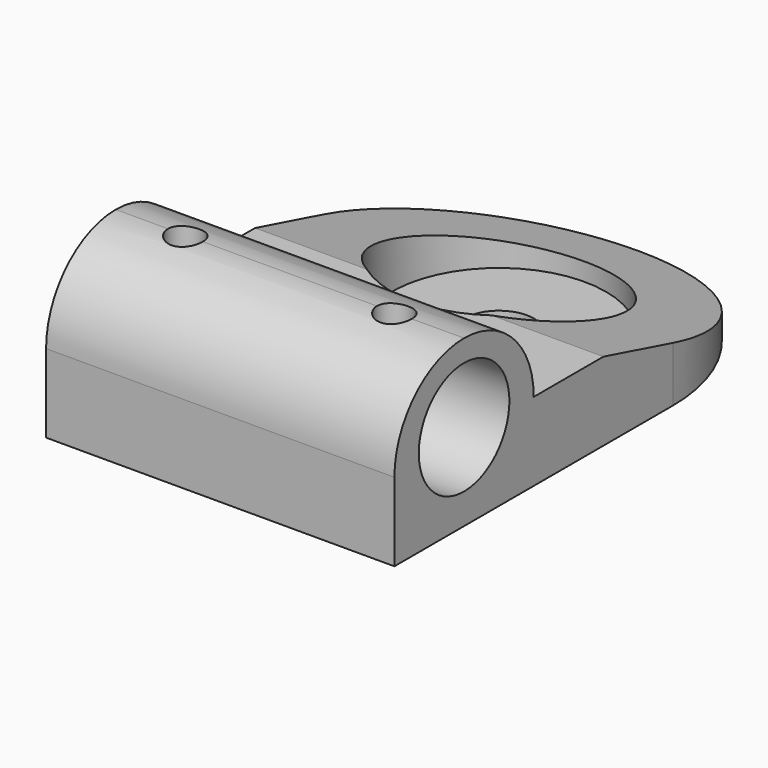
from build123d import *

# Parameters (mm, degrees)
F0_W         = 20
F0_H         = 30
F0_R         = 6.15
F1_DEPTH     = 4
F1_FACE_W    = 20
F1_FACE_H    = 30
F1_FACE_R    = 6.15
F0_R_2       = 2
F2_DEPTH     = 0.5
F3_W         = 20
F3_H         = 10
F4_DEPTH     = 5
F5_R         = 3.25
F6_DEPTH     = 25
F7_T1_DEPTH  = 97.9025398997
F8_R         = 9.99999
F9_R         = 1
F10_DEPTH    = 25
F11_T1_DEPTH = 45


# Not quite as in the source:
# - a fillet or chamfer that OpenCascade refuses, or shapes differently, is made with other operations: its cross-section is extruded or revolved along the edge and cut away or added
# - a fillet or chamfer is up to 0.001 mm smaller than in the source, because OpenCascade refuses the exact size
# - a feature names something its author has since deleted; it is built from what else it names


with BuildPart() as f1:
    # F0 (on Top) → F1 (new body)
    with BuildSketch(Plane.XY):
        with Locations((10, 15)):
            Rectangle(F0_W, F0_H)
        with Locations((10, 20)):
            Circle(F0_R, mode=Mode.SUBTRACT)
    extrude(amount=F1_DEPTH)

    # F1_face (on face) + F0 (on Top) → F2 (join)
    with BuildSketch(Plane(origin=(10, 13.7652894827, 4), x_dir=(1, 0, 0), z_dir=(0, 0, 1))):
        with Locations((0, 1.2347105173)):
            Rectangle(F1_FACE_W, F1_FACE_H)
        with Locations((0, 6.2347105173)):
            Circle(F1_FACE_R, mode=Mode.SUBTRACT)
    with BuildSketch(Plane.XY):
        with Locations((10, 20)):
            Circle(F0_R)
        with Locations((10, 20)):
            Circle(F0_R_2, mode=Mode.SUBTRACT)
    extrude(amount=F2_DEPTH)

    # F3 (on face) → F4 (join)
    with BuildSketch(Plane.XY.offset(4.5)):
        with Locations((10, 5)):
            Rectangle(F3_W, F3_H)
    extrude(amount=F4_DEPTH)

    # F5 (on face) → F6 (cut)
    with BuildSketch(Plane(origin=(0, 0, 0), x_dir=(0, -1, 0), z_dir=(-1, 0, 0))):
        with Locations((-5, 5)):
            Circle(F5_R)
    extrude(amount=-F6_DEPTH, mode=Mode.SUBTRACT)

    # F7: chamfer of 4 x 15 on 1 edges, made by hand

    # F7_s2 → F7_t1 (cut)
    with BuildSketch(Plane.YZ.offset(-38.9512699498)):
        Polygon((30, 0.5), (15, 4.5), (30, 4.5), align=None)
    extrude(amount=F7_T1_DEPTH, mode=Mode.SUBTRACT)

    # F8 (radius 10 in the source; OpenCascade refuses exactly that, so slightly less here)
    f8_edges = [f1.edges().sort_by_distance(p)[0] for p in [
        (0, 30, 0.25),
        (20, 30, 0.25),
    ]]
    fillet(f8_edges, radius=F8_R)

    # F9 (on face) → F10 (cut)
    with BuildSketch(Plane.XY.offset(9.5)):
        with Locations((4, 5)):
            Circle(F9_R)
        with Locations((16, 5)):
            Circle(F9_R)
    extrude(amount=-F10_DEPTH, mode=Mode.SUBTRACT)

    # F11: fillet of radius 5 on 2 edges, made by hand

    # F11_s2 → F11_t1 (cut)
    with BuildSketch(Plane.YZ.offset(-12.5)):
        with BuildLine():
            ThreePointArc((0, 4.5), (1.4644660941, 8.0355339059), (5, 9.5))
            Line((5, 9.5), (0, 9.5))
            Line((0, 9.5), (0, 4.5))
        make_face()
        with BuildLine():
            ThreePointArc((5, 9.5), (8.5355339059, 8.0355339059), (10, 4.5))
            Line((10, 4.5), (10, 9.5))
            Line((10, 9.5), (5, 9.5))
        make_face()
    extrude(amount=F11_T1_DEPTH, mode=Mode.SUBTRACT)


solid = f1.part
